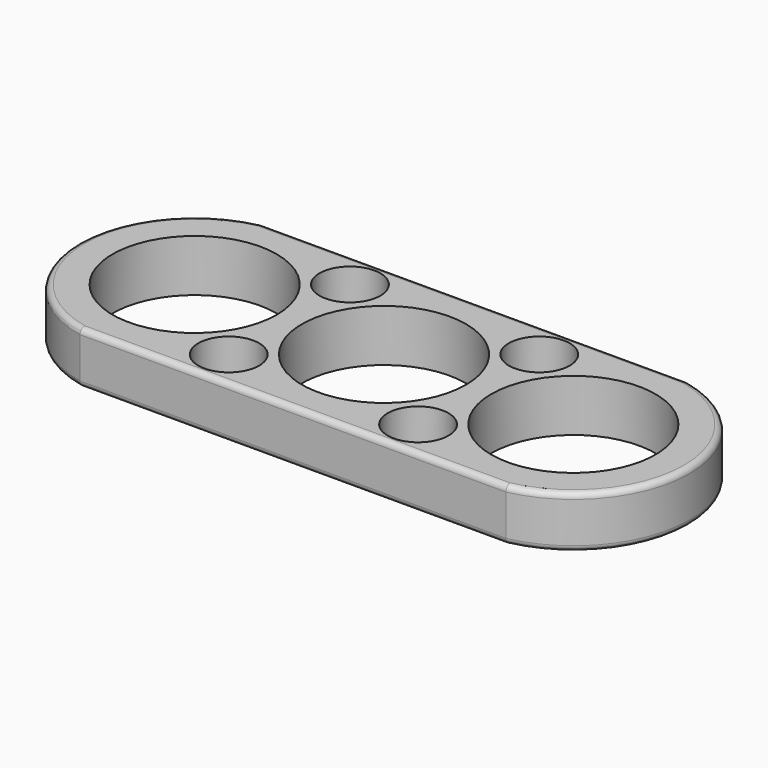
from build123d import *

# Parameters (mm, degrees)
F0_R        = 4.0800200383
F0_R_2      = 11.0109
F1_DEPTH    = 6.985
F2_T1_DEPTH = 63.627
F2_T4_ANGLE = 170.5132200492
F2_T6_ANGLE = 170.5132200492
F3_T1_DEPTH = 63.627
F3_T4_ANGLE = 170.5132200492
F3_T6_ANGLE = 170.5132200492


# Not quite as in the source:
# - a fillet or chamfer that OpenCascade refuses, or shapes differently, is made with other operations: its cross-section is extruded or revolved along the edge and cut away or added


with BuildPart() as f1:
    # F0 (on Top) → F1 (new body)
    with BuildSketch(Plane.XY):
        with BuildLine():
            Line((28.575, 15.2560200383), (-28.575, 15.2560200383))
            ThreePointArc((-28.575, 15.2560200383), (-40.9829, 0), (-28.575, -15.2560200383))
            Line((-28.575, -15.2560200383), (28.575, -15.2560200383))
            ThreePointArc((28.575, -15.2560200383), (40.9829, 0), (28.575, 15.2560200383))
        make_face()
        with Locations((-12.7, -10.16)):
            Circle(F0_R, mode=Mode.SUBTRACT)
        with Locations((12.7, -10.16)):
            Circle(F0_R, mode=Mode.SUBTRACT)
        with Locations((-25.4, 0)):
            Circle(F0_R_2, mode=Mode.SUBTRACT)
        with Locations((-12.7, 10.16)):
            Circle(F0_R, mode=Mode.SUBTRACT)
        with BuildLine():
            ThreePointArc((-11.0109, 0), (0, 11.0109), (11.0109, 0))
            ThreePointArc((11.0109, 0), (0, -11.0109), (-11.0109, 0))
        make_face(mode=Mode.SUBTRACT)
        with BuildLine():
            ThreePointArc((36.4109, 0), (25.4, -11.0109), (14.3891, 0))
            ThreePointArc((14.3891, 0), (25.4, 11.0109), (36.4109, 0))
        make_face(mode=Mode.SUBTRACT)
        with Locations((12.7, 10.16)):
            Circle(F0_R, mode=Mode.SUBTRACT)
    extrude(amount=F1_DEPTH)

    # F2: fillet of radius 0.762 on 4 edges, made by hand

    # F2_s2 → F2_t1 (cut)
    with BuildSketch(Plane.YZ.offset(-31.8135)):
        with BuildLine():
            ThreePointArc((-14.4940200383, 6.985), (-15.0328354056, 6.7618153673), (-15.2560200383, 6.223))
            Line((-15.2560200383, 6.223), (-15.2560200383, 6.985))
            Line((-15.2560200383, 6.985), (-14.4940200383, 6.985))
        make_face()
        with BuildLine():
            ThreePointArc((15.2560200383, 6.223), (15.0328354056, 6.7618153673), (14.4940200383, 6.985))
            Line((14.4940200383, 6.985), (15.2560200383, 6.985))
            Line((15.2560200383, 6.985), (15.2560200383, 6.223))
        make_face()
    extrude(amount=F2_T1_DEPTH, mode=Mode.SUBTRACT)

    # F2_s3 → F2_t4 (revolve, cut)
    with BuildSketch(Plane(origin=(-25.2263104474, -2.0932144122, 0), x_dir=(0, 0, 1), z_dir=(0.9965750492, 0.0826932365, 0))):
        with BuildLine():
            ThreePointArc((6.985, -16.921308207), (6.7618153673, -17.4601235742), (6.223, -17.683308207))
            Line((6.223, -17.683308207), (6.985, -17.683308207))
            Line((6.985, -17.683308207), (6.985, -16.921308207))
        make_face()
    revolve(axis=Axis((-25.4, 0, 6.985), (0, 0, 1)), revolution_arc=F2_T4_ANGLE, mode=Mode.SUBTRACT)

    # F2_s5 → F2_t6 (revolve, cut)
    with BuildSketch(Plane(origin=(25.2263104474, 2.0932144122, 0), x_dir=(0, 0, 1), z_dir=(-0.9965750492, -0.0826932365, 0))):
        with BuildLine():
            ThreePointArc((6.985, -16.921308207), (6.7618153673, -17.4601235742), (6.223, -17.683308207))
            Line((6.223, -17.683308207), (6.985, -17.683308207))
            Line((6.985, -17.683308207), (6.985, -16.921308207))
        make_face()
    revolve(axis=Axis((25.4, 0, 6.985), (0, 0, 1)), revolution_arc=F2_T6_ANGLE, mode=Mode.SUBTRACT)

    # F3: fillet of radius 0.762 on 4 edges, made by hand

    # F3_s2 → F3_t1 (cut)
    with BuildSketch(Plane.YZ.offset(-31.8135)):
        with BuildLine():
            ThreePointArc((15.2560200383, 0.762), (15.0328354056, 0.2231846327), (14.4940200383, 0))
            Line((14.4940200383, 0), (15.2560200383, 0))
            Line((15.2560200383, 0), (15.2560200383, 0.762))
        make_face()
        with BuildLine():
            ThreePointArc((-14.4940200383, 0), (-15.0328354056, 0.2231846327), (-15.2560200383, 0.762))
            Line((-15.2560200383, 0.762), (-15.2560200383, 0))
            Line((-15.2560200383, 0), (-14.4940200383, 0))
        make_face()
    extrude(amount=F3_T1_DEPTH, mode=Mode.SUBTRACT)

    # F3_s3 → F3_t4 (revolve, cut)
    with BuildSketch(Plane(origin=(-25.2263104474, -2.0932144122, 0), x_dir=(0, 0, 1), z_dir=(0.9965750492, 0.0826932365, 0))):
        with BuildLine():
            ThreePointArc((0, -16.921308207), (0.2231846327, -17.4601235742), (0.762, -17.683308207))
            Line((0.762, -17.683308207), (0, -17.683308207))
            Line((0, -17.683308207), (0, -16.921308207))
        make_face()
    revolve(axis=Axis((-25.4, 0, 0), (0, 0, 1)), revolution_arc=F3_T4_ANGLE, mode=Mode.SUBTRACT)

    # F3_s5 → F3_t6 (revolve, cut)
    with BuildSketch(Plane(origin=(25.2263104474, 2.0932144122, 0), x_dir=(0, 0, 1), z_dir=(-0.9965750492, -0.0826932365, 0))):
        with BuildLine():
            ThreePointArc((0, -16.921308207), (0.2231846327, -17.4601235742), (0.762, -17.683308207))
            Line((0.762, -17.683308207), (0, -17.683308207))
            Line((0, -17.683308207), (0, -16.921308207))
        make_face()
    revolve(axis=Axis((25.4, 0, 0), (0, 0, 1)), revolution_arc=F3_T6_ANGLE, mode=Mode.SUBTRACT)


solid = f1.part
